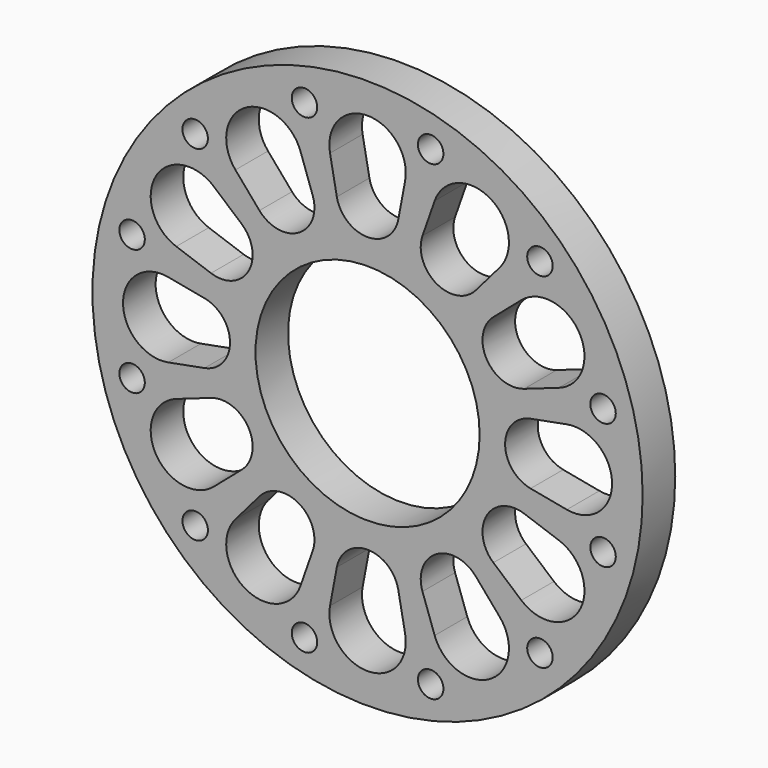
from build123d import *

# Parameters (mm, degrees)
F0_R     = 171.45
F0_R_2   = 7.9375
F0_R_3   = 69.85
F1_DEPTH = 25.4


# Not quite as in the source:
# - ends of sketch curves that miss each other by under 0.0002 mm in the source are joined


with BuildPart() as f1:
    # F0 (on Front) → F1 (new body)
    with BuildSketch(Plane.XZ):
        with Locations((-406.4, 317.5)):
            Circle(F0_R)
        with Locations((-513.8380376, 210.0619624)):
            Circle(F0_R_2, mode=Mode.SUBTRACT)
        with BuildLine():
            Line((-488.75442, 221.659196), (-473.7808914, 239.0848152))
            ThreePointArc((-473.7808914, 239.0848152), (-449.2625045681, 243.2599470835), (-440.6191192625, 219.9388323398))
            Line((-440.6191192625, 219.9388323398), (-448.2233606, 198.2585824))
            ThreePointArc((-448.2233606, 198.2585824), (-482.5999974139, 185.5177169793), (-488.75442, 221.659196))
        make_face(mode=Mode.SUBTRACT)
        with Locations((-553.1630796, 278.174958)):
            Circle(F0_R_2, mode=Mode.SUBTRACT)
        with BuildLine():
            Line((-525.6414176, 275.6766394), (-503.9611714, 283.2808914))
            ThreePointArc((-503.9611714, 283.2808914), (-480.6400529165, 274.6374954319), (-484.8151954053, 250.119120942))
            Line((-484.8151954053, 250.119120942), (-502.240804, 235.14558))
            ThreePointArc((-502.240804, 235.14558), (-538.3822830207, 241.3000025861), (-525.6414176, 275.6766394))
        make_face(mode=Mode.SUBTRACT)
        with Locations((-445.725042, 170.7369204)):
            Circle(F0_R_2, mode=Mode.SUBTRACT)
        with BuildLine():
            Line((-429.800639, 193.3222194), (-425.5459612, 215.9))
            ThreePointArc((-425.5459612, 215.9), (-406.4, 231.775), (-387.2540391788, 215.8999999286))
            Line((-387.2540391788, 215.8999999286), (-382.999361, 193.3222194))
            ThreePointArc((-382.999361, 193.3222194), (-406.4, 165.1), (-429.800639, 193.3222194))
        make_face(mode=Mode.SUBTRACT)
        with Locations((-367.074958, 170.7369204)):
            Circle(F0_R_2, mode=Mode.SUBTRACT)
        with BuildLine():
            Line((-364.5766394, 198.2585824), (-372.1808914, 219.9388286))
            ThreePointArc((-372.1808914, 219.9388286), (-363.5374954319, 243.2599470835), (-339.019120942, 239.0848045947))
            Line((-339.019120942, 239.0848045947), (-324.04558, 221.659196))
            ThreePointArc((-324.04558, 221.659196), (-330.2000025861, 185.5177169793), (-364.5766394, 198.2585824))
        make_face(mode=Mode.SUBTRACT)
        with Locations((-298.9619624, 210.0619624)):
            Circle(F0_R_2, mode=Mode.SUBTRACT)
        with BuildLine():
            Line((-310.559196, 235.14558), (-327.9848152, 250.1191086))
            ThreePointArc((-327.9848152, 250.1191086), (-332.1599470835, 274.6374954319), (-308.8388323398, 283.2808807375))
            Line((-308.8388323398, 283.2808807375), (-287.1585824, 275.6766394))
            ThreePointArc((-287.1585824, 275.6766394), (-274.4177169793, 241.3000025861), (-310.559196, 235.14558))
        make_face(mode=Mode.SUBTRACT)
        with Locations((-259.6369204, 278.174958)):
            Circle(F0_R_2, mode=Mode.SUBTRACT)
        with Locations((-553.1630796, 356.825042)):
            Circle(F0_R_2, mode=Mode.SUBTRACT)
        with BuildLine():
            Line((-530.5777806, 340.900639), (-508, 336.6459612))
            ThreePointArc((-508, 336.6459612), (-492.125, 317.5), (-508.0000000714, 298.3540391788))
            Line((-508.0000000714, 298.3540391788), (-530.5777806, 294.099361))
            ThreePointArc((-530.5777806, 294.099361), (-558.8, 317.5), (-530.5777806, 340.900639))
        make_face(mode=Mode.SUBTRACT)
        with BuildLine():
            Line((-502.240804, 399.85442), (-484.8151848, 384.8808914))
            ThreePointArc((-484.8151848, 384.8808914), (-480.6400529165, 360.3625045681), (-503.9611676602, 351.7191192625))
            Line((-503.9611676602, 351.7191192625), (-525.6414176, 359.3233606))
            ThreePointArc((-525.6414176, 359.3233606), (-538.3822830207, 393.6999974139), (-502.240804, 399.85442))
        make_face(mode=Mode.SUBTRACT)
        with Locations((-513.8380376, 424.9380376)):
            Circle(F0_R_2, mode=Mode.SUBTRACT)
        with BuildLine():
            Line((-448.2233606, 436.7414176), (-440.6191086, 415.0611714))
            ThreePointArc((-440.6191086, 415.0611714), (-449.2625045681, 391.7400529165), (-473.780879058, 395.9151954053))
            Line((-473.780879058, 395.9151954053), (-488.75442, 413.340804))
            ThreePointArc((-488.75442, 413.340804), (-482.5999974139, 449.4822830207), (-448.2233606, 436.7414176))
        make_face(mode=Mode.SUBTRACT)
        with Locations((-406.4, 317.5)):
            Circle(F0_R_3, mode=Mode.SUBTRACT)
        with BuildLine():
            Line((-382.999361, 441.6777806), (-387.2540388, 419.1))
            ThreePointArc((-387.2540388, 419.1), (-406.4, 403.225), (-425.5459608212, 419.1000000714))
            Line((-425.5459608212, 419.1000000714), (-429.800639, 441.6777806))
            ThreePointArc((-429.800639, 441.6777806), (-406.4, 469.9), (-382.999361, 441.6777806))
        make_face(mode=Mode.SUBTRACT)
        with BuildLine():
            Line((-324.04558, 413.340804), (-339.0191086, 395.9151848))
            ThreePointArc((-339.0191086, 395.9151848), (-363.5374954319, 391.7400529165), (-372.1808807375, 415.0611676602))
            Line((-372.1808807375, 415.0611676602), (-364.5766394, 436.7414176))
            ThreePointArc((-364.5766394, 436.7414176), (-330.2000025861, 449.4822830207), (-324.04558, 413.340804))
        make_face(mode=Mode.SUBTRACT)
        with Locations((-445.725042, 464.2630796)):
            Circle(F0_R_2, mode=Mode.SUBTRACT)
        with Locations((-367.074958, 464.2630796)):
            Circle(F0_R_2, mode=Mode.SUBTRACT)
        with BuildLine():
            Line((-282.2222194, 294.099361), (-304.8, 298.3540388))
            ThreePointArc((-304.8, 298.3540388), (-320.675, 317.5), (-304.7999999286, 336.6459608212))
            Line((-304.7999999286, 336.6459608212), (-282.2222194, 340.900639))
            ThreePointArc((-282.2222194, 340.900639), (-254, 317.5), (-282.2222194, 294.099361))
        make_face(mode=Mode.SUBTRACT)
        with BuildLine():
            Line((-287.1585824, 359.3233606), (-308.8388286, 351.7191086))
            ThreePointArc((-308.8388286, 351.7191086), (-332.1599470835, 360.3625045681), (-327.9848045947, 384.880879058))
            Line((-327.9848045947, 384.880879058), (-310.559196, 399.85442))
            ThreePointArc((-310.559196, 399.85442), (-274.4177169793, 393.6999974139), (-287.1585824, 359.3233606))
        make_face(mode=Mode.SUBTRACT)
        with Locations((-259.6369204, 356.825042)):
            Circle(F0_R_2, mode=Mode.SUBTRACT)
        with Locations((-298.9619624, 424.9380376)):
            Circle(F0_R_2, mode=Mode.SUBTRACT)
    extrude(amount=F1_DEPTH)


solid = f1.part
